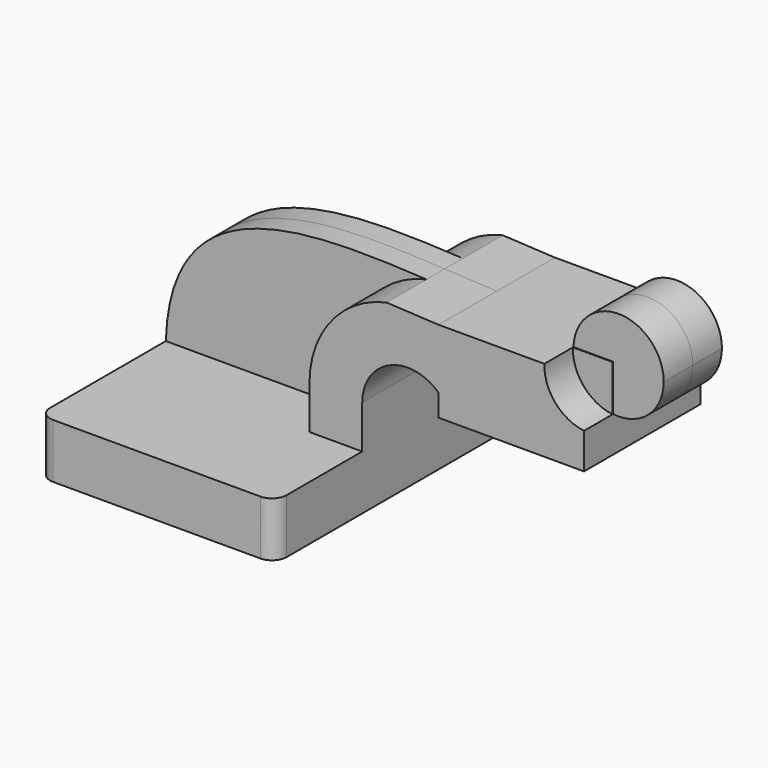
from build123d import *

# Parameters (mm, degrees)
F1_DEPTH = 63.5
F2_DEPTH = 25.4
F3_DEPTH = 7.9375
F4_R     = 5.08
F5_DEPTH = 12.7
F6_DEPTH = 12.954


# Not quite as in the source:
# - a feature names something its author has since deleted; it is built from what else it names


with BuildPart() as f1:
    # F0 (on Front) → F1 (new body, symmetric)
    with BuildSketch(Plane.XZ):
        Polygon((41.275, -9.525), (41.275, 9.525), (22.86, 9.525), (-41.275, 9.525), (-41.275, -9.525), align=None)
    extrude(amount=F1_DEPTH, both=True)

    # F0 (on Front) → F2 (join, symmetric)
    with BuildSketch(Plane.XZ):
        with BuildLine():
            Line((22.86, 9.525), (41.275, 9.525))
            Line((41.275, 9.525), (41.275, 24.6097946961))
            ThreePointArc((41.275, 24.6097946961), (50.7878547404, 39.1541658648), (67.925549001, 36.2675461399))
            Line((67.925549001, 36.2675461399), (67.925549001, 57.1627))
            add(Edge.make_bspline(
                [(49.7285614833, 58.0870459324), (56.0365853953, 57.7436105447), (62.1682234861, 57.3725135069), (67.925549001, 57.1627)],
                knots=[103.2417964532, 103.2417964532, 103.2417964532, 103.2417964532, 119.139037949, 119.139037949, 119.139037949, 119.139037949], degree=3))
            ThreePointArc((49.7285614833, 58.0870459324), (30.4078494999, 46.0728207323), (22.86, 24.6097946961))
            Line((22.86, 24.6097946961), (22.86, 9.525))
        make_face()
        with BuildLine():
            Line((67.925549001, 57.1627), (67.925549001, 36.2675461399))
            Line((67.925549001, 36.2675461399), (67.925549001, 28.5877))
            Line((67.925549001, 28.5877), (118.725549001, 28.5877))
            Line((118.725549001, 28.5877), (118.725549001, 41.0749236981))
            ThreePointArc((118.725549001, 41.0749236981), (108.6814992651, 46.435602827), (104.8671576362, 57.1627))
            Line((104.8671576362, 57.1627), (67.925549001, 57.1627))
        make_face()
    extrude(amount=F2_DEPTH, both=True)

    # F0 (on Front) → F3 (join, symmetric)
    with BuildSketch(Plane.XZ):
        with BuildLine():
            Line((-41.275, 9.525), (22.86, 9.525))
            Line((22.86, 9.525), (22.86, 24.6097946961))
            ThreePointArc((22.86, 24.6097946961), (30.4078494999, 46.0728207323), (49.7285614833, 58.0870459324))
            add(Edge.make_bspline(
                [(-41.275, 9.525), (-39.6433941578, 61.3811419555), (8.7622264795, 60.3174257381), (49.7285614833, 58.0870459324)],
                knots=[0, 0, 0, 0, 103.2417964532, 103.2417964532, 103.2417964532, 103.2417964532], degree=3))
        make_face()
    extrude(amount=F3_DEPTH, both=True)

    # F4
    f4_edges = [f1.edges().sort_by_distance(p)[0] for p in [
        (-41.275, -63.5, 0),
        (41.275, -63.5, 0),
        (41.275, 63.5, 0),
        (-41.275, 63.5, 0),
    ]]
    fillet(f4_edges, radius=F4_R)


with BuildPart() as f5:
    # F0 (on Front) → F5 (new body, symmetric)
    with BuildSketch(Plane.XZ):
        with BuildLine():
            ThreePointArc((136.389559184, 56.7242838442), (120.8445389242, 72.4870089264), (104.8671576362, 57.1627))
            Line((104.8671576362, 57.1627), (118.725549001, 57.1627))
            Line((118.725549001, 57.1627), (118.725549001, 41.0749236981))
            ThreePointArc((118.725549001, 41.0749236981), (131.0790951476, 44.9247104544), (136.389559184, 56.7242838442))
        make_face()
    extrude(amount=F5_DEPTH, both=True)


with BuildPart() as f6:
    # F0 (on Front) → F6 (new body, symmetric)
    with BuildSketch(Plane.XZ):
        with BuildLine():
            Line((118.725549001, 57.1627), (104.8671576362, 57.1627))
            ThreePointArc((104.8671576362, 57.1627), (108.6814992651, 46.435602827), (118.725549001, 41.0749236981))
            Line((118.725549001, 41.0749236981), (118.725549001, 57.1627))
        make_face()
    extrude(amount=F6_DEPTH, both=True)


solid = Compound([f1.part, f5.part, f6.part])
